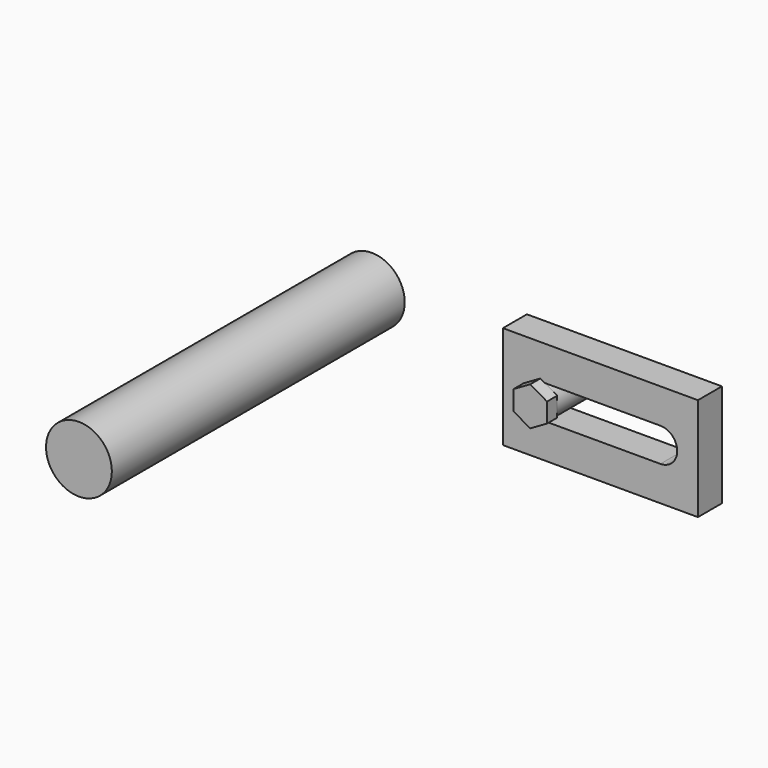
from build123d import *

# Parameters (mm, degrees)
F0_W     = 165.1000029331
F0_H     = 87.1681807961
F1_DEPTH = 25.4
F3_DEPTH = 10.80206
F5_DEPTH = 50.8
F6_R     = 27.8649500895
F7_DEPTH = 309.9365


with BuildPart() as f1:
    # F0 (on Front) → F1 (new body)
    with BuildSketch(Plane.XZ):
        Rectangle(F0_W, F0_H)
        with BuildLine():
            ThreePointArc((-50.8, -14.2267111767), (-65.0267111767, 0), (-50.8, 14.2267111767))
            Line((-50.8, 14.2267111767), (50.8, 14.2267111767))
            ThreePointArc((50.8, 14.2267111767), (65.0267111767, 0), (50.8, -14.2267111767))
            Line((50.8, -14.2267111767), (-50.8, -14.2267111767))
        make_face(mode=Mode.SUBTRACT)
    extrude(amount=F1_DEPTH)


with BuildPart() as f3:
    # F2 (on face) → F3 (new body)
    with BuildSketch(Plane.XZ.offset(25.4)):
        Polygon((-65.0267111767, 8.2137955275), (-65.0267111767, -8.2137955275), (-50.8, -16.4275910551), (-36.5732888233, -8.2137955275), (-36.5732888233, 8.2137955275), (-50.8, 16.4275910551), align=None)
    extrude(amount=F3_DEPTH)

    # F4 (on face) → F5 (join)
    with BuildSketch(Plane(origin=(0, -25.4, 0), x_dir=(-1, 0, 0), z_dir=(0, 1, 0))):
        with BuildLine():
            ThreePointArc((50.8, -14.2267111767), (65.0267111767, 0), (50.8, 14.2267111767))
            ThreePointArc((50.8, 14.2267111767), (36.5732888233, 0), (50.8, -14.2267111767))
        make_face()
    extrude(amount=F5_DEPTH)


with BuildPart() as f7:
    # F6 (on Front) → F7 (new body)
    with BuildSketch(Plane.XZ):
        with Locations((-213.837787509, 18.8797675073)):
            Circle(F6_R)
    extrude(amount=F7_DEPTH)


solid = Compound([f1.part, f3.part, f7.part])
